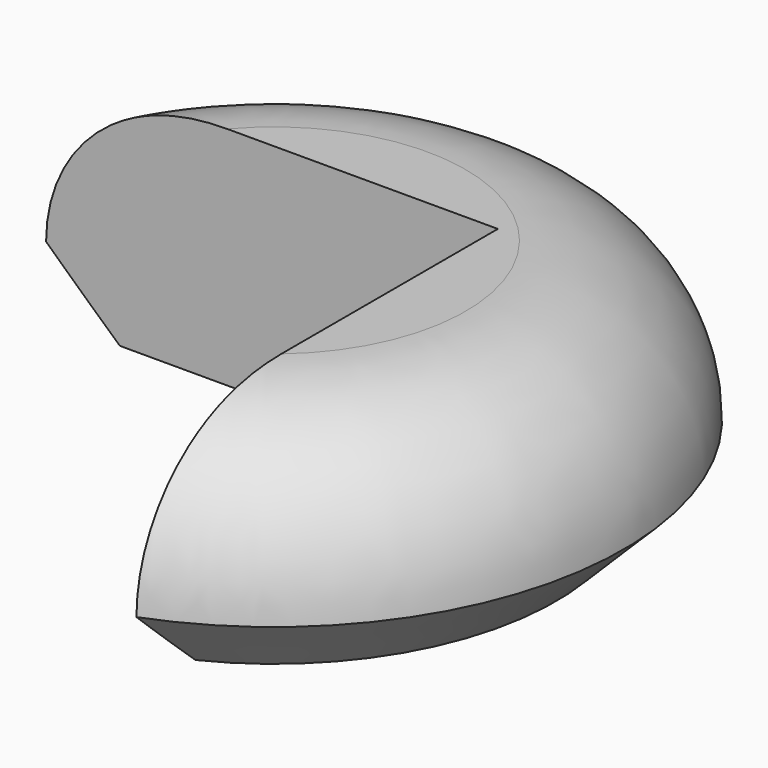
from build123d import *

# Parameters (mm, degrees)
F1_DEPTH = 10
F2_R     = 7
F3_SIZE  = 2.99999


# Not quite as in the source:
# - a fillet or chamfer is up to 0.001 mm smaller than in the source, because OpenCascade refuses the exact size


with BuildPart() as f1:
    # F0 (on Top) → F1 (new body)
    with BuildSketch(Plane.XY):
        with BuildLine():
            Line((-20, 0), (0, 0))
            Line((0, 0), (0, -20))
            ThreePointArc((0, -20), (5.4462447196, 5.4462447196), (-20, 0))
        make_face()
    extrude(amount=F1_DEPTH)

    # F2
    f2_edges = [f1.edges().sort_by_distance(p)[0] for p in [
        (5.446245, 5.446245, 10),
    ]]
    fillet(f2_edges, radius=F2_R)

    # F3 (size 3 in the source; OpenCascade refuses exactly that, so slightly less here)
    f3_edges = [f1.edges().sort_by_distance(p)[0] for p in [
        (5.446245, 5.446245, 0),
    ]]
    chamfer(f3_edges, length=F3_SIZE)


solid = f1.part
